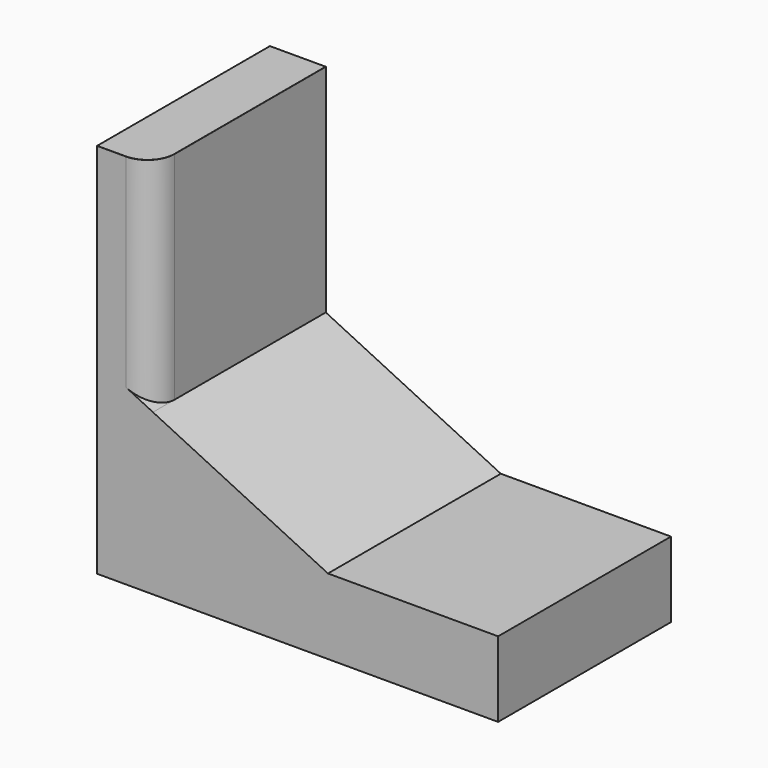
from build123d import *

# Parameters (mm, degrees)
F1_DEPTH    = 40
F2_R        = 0.0241421356
F3_T2_ANGLE = 90
F3_T6_DEPTH = 52.5499999523


# Not quite as in the source:
# - a fillet or chamfer that OpenCascade refuses, or shapes differently, is made with other operations: its cross-section is extruded or revolved along the edge and cut away or added


with BuildPart() as f1:
    # F0 (on Front) → F1 (new body)
    with BuildSketch(Plane.XZ):
        Polygon((0, 40.0499999523), (0, 0), (0, -29.6999998391), (74.2500051856, -29.6999998391), (74.2500051856, -15.7500002533), (42.7500009537, -15.7500002533), (10.349996388, 0), (10.349996388, 40.0499999523), align=None)
    extrude(amount=F1_DEPTH)

    # F2
    f2_edges = [f1.edges().sort_by_distance(p)[0] for p in [
        (10.349996, -20, 40.05),
        (0, -20, 40.05),
        (5.174998, 0, 40.05),
        (5.174998, -40, 40.05),
    ]]
    fillet(f2_edges, radius=F2_R)

    # F3: fillet of radius 5 on 5 edges, made by hand

    # F3_s1 → F3_t2 (revolve, cut)
    with BuildSketch(Plane.YZ.offset(5.349996388)):
        with BuildLine():
            ThreePointArc((-39.9758578644, 40.0499999523), (-39.9929289322, 40.0429288845), (-40, 40.0258578167))
            Line((-40, 40.0258578167), (-40, 40.0499999523))
            Line((-40, 40.0499999523), (-39.9758578644, 40.0499999523))
        make_face()
    revolve(axis=Axis((5.349996388, -35, 40.0499999523), (0, 0, 1)), revolution_arc=F3_T2_ANGLE, mode=Mode.SUBTRACT)


with BuildPart() as f3_tool4:
    # F3_s5 → F3_t6 (new body)
    with BuildSketch(Plane.XY.offset(-12.5)):
        with BuildLine():
            ThreePointArc((10.349996388, -35), (8.8855302939, -38.5355339059), (5.349996388, -40))
            Line((5.349996388, -40), (10.349996388, -40))
            Line((10.349996388, -40), (10.349996388, -35))
        make_face()
    extrude(amount=F3_T6_DEPTH)

    split(bisect_by=Plane(origin=(1.9782716516, 0, 4.0695879055), x_dir=(0, 1, 0), z_dir=(0.4371926627, 0, 0.8993678756)), keep=Keep.TOP)


with BuildPart() as f1_1:
    add(f1.part)

    # F3_t3: cut F3_tool4
    add(f3_tool4.part, mode=Mode.SUBTRACT)


solid = f1_1.part
